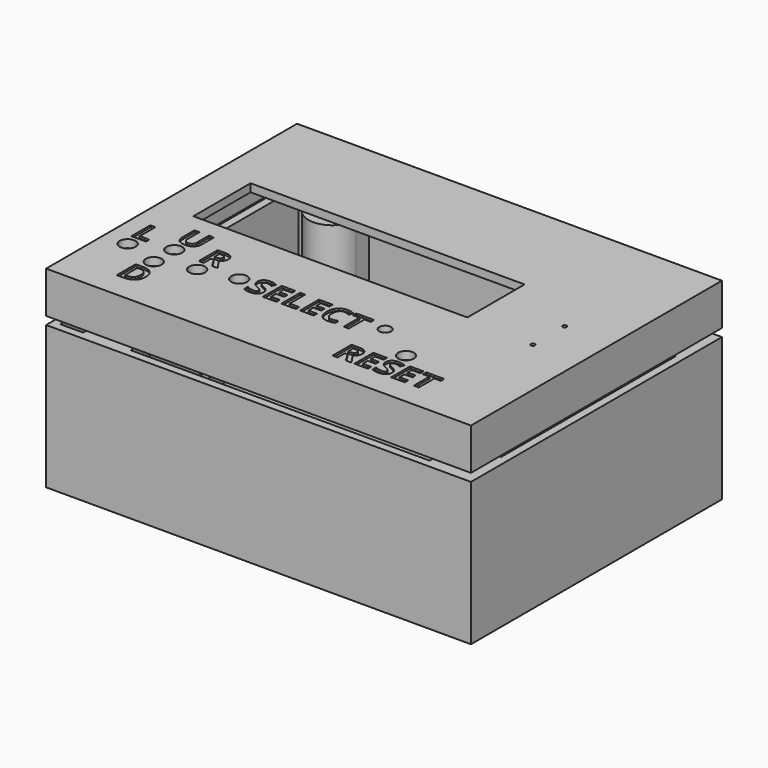
from build123d import *
from build123d import SkipClean  # not in build123d's __all__

# Parameters (mm, degrees)
F3_W         = 2
F3_H         = 5.75
F3_H_2       = 3.5
F3_R         = 2.1844
F3_H_3       = 10.1
F3_H_4       = 11
F4_DEPTH     = 2
F5_DEPTH     = 34
F6_START     = 3
F6_DEPTH     = 4
F7_START     = 3
F7_DEPTH     = 13
F8_START     = 32
F3_R_2       = 2
F8_DEPTH     = 2
F10_START    = 44.5
F9_W         = 107
F9_H         = 79
F9_R         = 0.5
F9_R_2       = 2.7813
F9_TEXT_SIZE = 8.3333333333
F10_DEPTH    = 2
F11_START    = 36
F11_DEPTH    = 8.5
F2_W         = 69
F2_H         = 18
F2_R         = 2
F2_R_2       = 1.5
F12_DEPTH    = 46.501
F13_START    = 46
F13_DEPTH    = 0.5
F14_R        = 2.75
F14_R_2      = 1.75
F15_DEPTH    = 7
F16_DEPTH    = 11.5


# Not quite as in the source:
# - after a boolean that leaves OpenCascade's solid faulty, fix() repairs it
# - a feature names something its author has since deleted; it is built from what else it names
# - Text() gives the source's letters only with a copy of the font that has no kerning and outlines rounded to 1/6400 em; it was checked with that copy


with BuildPart() as f4:
    # F3 (on Top) → F4 (new body)
    with BuildSketch(Plane.XY):
        Polygon((-51.5, 16.58), (-51.5, 37.5), (-45.8, 37.5), (-39.8, 37.5), (-33.8, 37.5), (41.5, 37.5), (47.5, 37.5), (51.5, 37.5), (51.5, 33.5), (51.5, 27.5), (51.5, -27.5), (51.5, -33.5), (51.5, -37.5), (47.4999999936, -37.5), (41.5, -37.5), (-33.8, -37.5), (-39.8, -37.5), (-45.8, -37.5), (-51.5, -37.5), (-51.5, -23.87), (-53.5, -23.87), (-53.5, -39.5), (53.5, -39.5), (53.5, 39.5), (-53.5, 39.5), (-53.5, 16.58), align=None)
        with Locations((-52.5, 3.605)):
            Rectangle(F3_W, F3_H)
        with Locations((-52.5, -11.12)):
            Rectangle(F3_W, F3_H_2)
        with BuildLine():
            Line((-45.8, 37.5), (-51.5, 37.5))
            Line((-51.5, 37.5), (-51.5, 16.58))
            Line((-51.5, 16.58), (-51.5, 6.48))
            Line((-51.5, 6.48), (-51.5, 0.73))
            Line((-51.5, 0.73), (-51.5, -9.37))
            Line((-51.5, -9.37), (-51.5, -12.87))
            Line((-51.5, -12.87), (-51.5, -23.87))
            Line((-51.5, -23.87), (-51.5, -37.5))
            Line((-51.5, -37.5), (-45.8, -37.5))
            Line((-45.8, -37.5), (-45.8, -33.5))
            ThreePointArc((-45.8, -33.5), (-39.8, -27.5), (-33.8, -33.5))
            Line((-33.8, -33.5), (-33.8, -37.5))
            Line((-33.8, -37.5), (41.5, -37.5))
            Line((41.5, -37.5), (41.5, -33.5))
            ThreePointArc((41.5, -33.5), (43.2573593129, -29.2573593129), (47.5, -27.5))
            Line((47.5, -27.5), (51.5, -27.5))
            Line((51.5, -27.5), (51.5, 27.5))
            Line((51.5, 27.5), (47.5, 27.5))
            ThreePointArc((47.5, 27.5), (43.2573593129, 29.2573593129), (41.5, 33.5))
            Line((41.5, 33.5), (41.5, 37.5))
            Line((41.5, 37.5), (-33.8, 37.5))
            Line((-33.8, 37.5), (-33.8, 33.5))
            ThreePointArc((-33.8, 33.5), (-39.8, 27.5), (-45.8, 33.5))
            Line((-45.8, 33.5), (-45.8, 37.5))
        make_face()
        with Locations((-35.56, -24.13)):
            Circle(F3_R, mode=Mode.SUBTRACT)
        with Locations((46.99, -24.13)):
            Circle(F3_R, mode=Mode.SUBTRACT)
        with Locations((-35.56, 24.13)):
            Circle(F3_R, mode=Mode.SUBTRACT)
        with Locations((-52.5, 11.53)):
            Rectangle(F3_W, F3_H_3)
        with Locations((-52.5, -4.32)):
            Rectangle(F3_W, F3_H_3)
        with Locations((-52.5, -18.37)):
            Rectangle(F3_W, F3_H_4)
        with BuildLine():
            Line((-45.8, 37.5), (-51.5, 37.5))
            Line((-51.5, 37.5), (-51.5, 16.58))
            Line((-51.5, 16.58), (-51.5, 6.48))
            Line((-51.5, 6.48), (-51.5, 0.73))
            Line((-51.5, 0.73), (-51.5, -9.37))
            Line((-51.5, -9.37), (-51.5, -12.87))
            Line((-51.5, -12.87), (-51.5, -23.87))
            Line((-51.5, -23.87), (-51.5, -37.5))
            Line((-51.5, -37.5), (-45.8, -37.5))
            Line((-45.8, -37.5), (-45.8, -33.5))
            ThreePointArc((-45.8, -33.5), (-39.8, -27.5), (-33.8, -33.5))
            Line((-33.8, -33.5), (-33.8, -37.5))
            Line((-33.8, -37.5), (41.5, -37.5))
            Line((41.5, -37.5), (41.5, -33.5))
            ThreePointArc((41.5, -33.5), (43.2573593129, -29.2573593129), (47.5, -27.5))
            Line((47.5, -27.5), (51.5, -27.5))
            Line((51.5, -27.5), (51.5, 27.5))
            Line((51.5, 27.5), (47.5, 27.5))
            ThreePointArc((47.5, 27.5), (43.2573593129, 29.2573593129), (41.5, 33.5))
            Line((41.5, 33.5), (41.5, 37.5))
            Line((41.5, 37.5), (-33.8, 37.5))
            Line((-33.8, 37.5), (-33.8, 33.5))
            ThreePointArc((-33.8, 33.5), (-39.8, 27.5), (-45.8, 33.5))
            Line((-45.8, 33.5), (-45.8, 37.5))
        make_face()
        with Locations((-35.56, -24.13)):
            Circle(F3_R, mode=Mode.SUBTRACT)
        with Locations((46.99, -24.13)):
            Circle(F3_R, mode=Mode.SUBTRACT)
        with Locations((-35.56, 24.13)):
            Circle(F3_R, mode=Mode.SUBTRACT)
        with BuildLine():
            Line((-45.8, -33.5), (-45.8, -37.5))
            Line((-45.8, -37.5), (-39.8, -37.5))
            Line((-39.8, -37.5), (-33.8, -37.5))
            Line((-33.8, -37.5), (-33.8, -33.5))
            ThreePointArc((-33.8, -33.5), (-39.8, -27.5), (-45.8, -33.5))
        make_face()
        with BuildLine():
            ThreePointArc((-35.8, -33.5), (-36.9715728753, -36.3284271247), (-39.8, -37.5))
            ThreePointArc((-39.8, -37.5), (-42.6284271247, -30.6715728753), (-35.8, -33.5))
        make_face(mode=Mode.SUBTRACT)
        with BuildLine():
            Line((-45.8, -33.5), (-45.8, -37.5))
            Line((-45.8, -37.5), (-39.8, -37.5))
            Line((-39.8, -37.5), (-33.8, -37.5))
            Line((-33.8, -37.5), (-33.8, -33.5))
            ThreePointArc((-33.8, -33.5), (-39.8, -27.5), (-45.8, -33.5))
        make_face()
        with BuildLine():
            ThreePointArc((-35.8, -33.5), (-36.9715728753, -36.3284271247), (-39.8, -37.5))
            ThreePointArc((-39.8, -37.5), (-42.6284271247, -30.6715728753), (-35.8, -33.5))
        make_face(mode=Mode.SUBTRACT)
        with BuildLine():
            Line((-45.8, 37.5), (-51.5, 37.5))
            Line((-51.5, 37.5), (-51.5, 16.58))
            Line((-51.5, 16.58), (-51.5, 6.48))
            Line((-51.5, 6.48), (-51.5, 0.73))
            Line((-51.5, 0.73), (-51.5, -9.37))
            Line((-51.5, -9.37), (-51.5, -12.87))
            Line((-51.5, -12.87), (-51.5, -23.87))
            Line((-51.5, -23.87), (-51.5, -37.5))
            Line((-51.5, -37.5), (-45.8, -37.5))
            Line((-45.8, -37.5), (-45.8, -33.5))
            ThreePointArc((-45.8, -33.5), (-39.8, -27.5), (-33.8, -33.5))
            Line((-33.8, -33.5), (-33.8, -37.5))
            Line((-33.8, -37.5), (41.5, -37.5))
            Line((41.5, -37.5), (41.5, -33.5))
            ThreePointArc((41.5, -33.5), (43.2573593129, -29.2573593129), (47.5, -27.5))
            Line((47.5, -27.5), (51.5, -27.5))
            Line((51.5, -27.5), (51.5, 27.5))
            Line((51.5, 27.5), (47.5, 27.5))
            ThreePointArc((47.5, 27.5), (43.2573593129, 29.2573593129), (41.5, 33.5))
            Line((41.5, 33.5), (41.5, 37.5))
            Line((41.5, 37.5), (-33.8, 37.5))
            Line((-33.8, 37.5), (-33.8, 33.5))
            ThreePointArc((-33.8, 33.5), (-39.8, 27.5), (-45.8, 33.5))
            Line((-45.8, 33.5), (-45.8, 37.5))
        make_face()
        with Locations((-35.56, -24.13)):
            Circle(F3_R, mode=Mode.SUBTRACT)
        with Locations((46.99, -24.13)):
            Circle(F3_R, mode=Mode.SUBTRACT)
        with Locations((-35.56, 24.13)):
            Circle(F3_R, mode=Mode.SUBTRACT)
        with BuildLine():
            Line((-39.8, 37.5), (-45.8, 37.5))
            Line((-45.8, 37.5), (-45.8, 33.5))
            ThreePointArc((-45.8, 33.5), (-39.8, 27.5), (-33.8, 33.5))
            Line((-33.8, 33.5), (-33.8, 37.5))
            Line((-33.8, 37.5), (-39.8, 37.5))
        make_face()
        with BuildLine():
            ThreePointArc((-35.8, 33.5), (-42.6284271247, 30.6715728753), (-39.8, 37.5))
            ThreePointArc((-39.8, 37.5), (-36.9715728753, 36.3284271247), (-35.8, 33.5))
        make_face(mode=Mode.SUBTRACT)
        with BuildLine():
            Line((47.5, 37.5), (41.5, 37.5))
            Line((41.5, 37.5), (41.5, 33.5))
            ThreePointArc((41.5, 33.5), (43.2573593129, 29.2573593129), (47.5, 27.5))
            Line((47.5, 27.5), (51.5, 27.5))
            Line((51.5, 27.5), (51.5, 33.5))
            ThreePointArc((51.5, 33.5), (44.6715728753, 30.6715728753), (47.5, 37.5))
        make_face()
        with BuildLine():
            Line((51.5, -33.5), (51.5, -27.5))
            Line((51.5, -27.5), (47.5, -27.5))
            ThreePointArc((47.5, -27.5), (43.2573593129, -29.2573593129), (41.5, -33.5))
            Line((41.5, -33.5), (41.5, -37.5))
            Line((41.5, -37.5), (47.4999999936, -37.5))
            ThreePointArc((47.4999999936, -37.5), (44.6715728775, -30.671572873), (51.5, -33.5))
        make_face()
        with BuildLine():
            Line((51.5, -37.5), (51.5, -33.5))
            ThreePointArc((51.5, -33.5), (50.3284271225, -36.328427127), (47.4999999936, -37.5))
            Line((47.4999999936, -37.5), (51.5, -37.5))
        make_face()
        with BuildLine():
            Line((-39.8, 37.5), (-45.8, 37.5))
            Line((-45.8, 37.5), (-45.8, 33.5))
            ThreePointArc((-45.8, 33.5), (-39.8, 27.5), (-33.8, 33.5))
            Line((-33.8, 33.5), (-33.8, 37.5))
            Line((-33.8, 37.5), (-39.8, 37.5))
        make_face()
        with BuildLine():
            ThreePointArc((-35.8, 33.5), (-42.6284271247, 30.6715728753), (-39.8, 37.5))
            ThreePointArc((-39.8, 37.5), (-36.9715728753, 36.3284271247), (-35.8, 33.5))
        make_face(mode=Mode.SUBTRACT)
        with BuildLine():
            Line((51.5, 37.5), (47.5, 37.5))
            ThreePointArc((47.5, 37.5), (50.3284271247, 36.3284271247), (51.5, 33.5))
            Line((51.5, 33.5), (51.5, 37.5))
        make_face()
    extrude(amount=-F4_DEPTH)

    # F3 (on Top) → F5 (join)
    with BuildSketch(Plane.XY):
        Polygon((-51.5, 16.58), (-51.5, 37.5), (-45.8, 37.5), (-39.8, 37.5), (-33.8, 37.5), (41.5, 37.5), (47.5, 37.5), (51.5, 37.5), (51.5, 33.5), (51.5, 27.5), (51.5, -27.5), (51.5, -33.5), (51.5, -37.5), (47.4999999936, -37.5), (41.5, -37.5), (-33.8, -37.5), (-39.8, -37.5), (-45.8, -37.5), (-51.5, -37.5), (-51.5, -23.87), (-53.5, -23.87), (-53.5, -39.5), (53.5, -39.5), (53.5, 39.5), (-53.5, 39.5), (-53.5, 16.58), align=None)
        with Locations((-52.5, -11.12)):
            Rectangle(F3_W, F3_H_2)
        with Locations((-52.5, 3.605)):
            Rectangle(F3_W, F3_H)
        with BuildLine():
            Line((-39.8, 37.5), (-45.8, 37.5))
            Line((-45.8, 37.5), (-45.8, 33.5))
            ThreePointArc((-45.8, 33.5), (-39.8, 27.5), (-33.8, 33.5))
            Line((-33.8, 33.5), (-33.8, 37.5))
            Line((-33.8, 37.5), (-39.8, 37.5))
        make_face()
        with BuildLine():
            ThreePointArc((-35.8, 33.5), (-42.6284271247, 30.6715728753), (-39.8, 37.5))
            ThreePointArc((-39.8, 37.5), (-36.9715728753, 36.3284271247), (-35.8, 33.5))
        make_face(mode=Mode.SUBTRACT)
        with BuildLine():
            Line((-39.8, 37.5), (-45.8, 37.5))
            Line((-45.8, 37.5), (-45.8, 33.5))
            ThreePointArc((-45.8, 33.5), (-39.8, 27.5), (-33.8, 33.5))
            Line((-33.8, 33.5), (-33.8, 37.5))
            Line((-33.8, 37.5), (-39.8, 37.5))
        make_face()
        with BuildLine():
            ThreePointArc((-35.8, 33.5), (-42.6284271247, 30.6715728753), (-39.8, 37.5))
            ThreePointArc((-39.8, 37.5), (-36.9715728753, 36.3284271247), (-35.8, 33.5))
        make_face(mode=Mode.SUBTRACT)
        with BuildLine():
            Line((47.5, 37.5), (41.5, 37.5))
            Line((41.5, 37.5), (41.5, 33.5))
            ThreePointArc((41.5, 33.5), (43.2573593129, 29.2573593129), (47.5, 27.5))
            Line((47.5, 27.5), (51.5, 27.5))
            Line((51.5, 27.5), (51.5, 33.5))
            ThreePointArc((51.5, 33.5), (44.6715728753, 30.6715728753), (47.5, 37.5))
        make_face()
        with BuildLine():
            Line((51.5, 37.5), (47.5, 37.5))
            ThreePointArc((47.5, 37.5), (50.3284271247, 36.3284271247), (51.5, 33.5))
            Line((51.5, 33.5), (51.5, 37.5))
        make_face()
        with BuildLine():
            Line((-45.8, -33.5), (-45.8, -37.5))
            Line((-45.8, -37.5), (-39.8, -37.5))
            Line((-39.8, -37.5), (-33.8, -37.5))
            Line((-33.8, -37.5), (-33.8, -33.5))
            ThreePointArc((-33.8, -33.5), (-39.8, -27.5), (-45.8, -33.5))
        make_face()
        with BuildLine():
            ThreePointArc((-35.8, -33.5), (-36.9715728753, -36.3284271247), (-39.8, -37.5))
            ThreePointArc((-39.8, -37.5), (-42.6284271247, -30.6715728753), (-35.8, -33.5))
        make_face(mode=Mode.SUBTRACT)
        with BuildLine():
            Line((-45.8, -33.5), (-45.8, -37.5))
            Line((-45.8, -37.5), (-39.8, -37.5))
            Line((-39.8, -37.5), (-33.8, -37.5))
            Line((-33.8, -37.5), (-33.8, -33.5))
            ThreePointArc((-33.8, -33.5), (-39.8, -27.5), (-45.8, -33.5))
        make_face()
        with BuildLine():
            ThreePointArc((-35.8, -33.5), (-36.9715728753, -36.3284271247), (-39.8, -37.5))
            ThreePointArc((-39.8, -37.5), (-42.6284271247, -30.6715728753), (-35.8, -33.5))
        make_face(mode=Mode.SUBTRACT)
        with BuildLine():
            Line((51.5, -37.5), (51.5, -33.5))
            ThreePointArc((51.5, -33.5), (50.3284271225, -36.328427127), (47.4999999936, -37.5))
            Line((47.4999999936, -37.5), (51.5, -37.5))
        make_face()
        with BuildLine():
            Line((51.5, -33.5), (51.5, -27.5))
            Line((51.5, -27.5), (47.5, -27.5))
            ThreePointArc((47.5, -27.5), (43.2573593129, -29.2573593129), (41.5, -33.5))
            Line((41.5, -33.5), (41.5, -37.5))
            Line((41.5, -37.5), (47.4999999936, -37.5))
            ThreePointArc((47.4999999936, -37.5), (44.6715728775, -30.671572873), (51.5, -33.5))
        make_face()
        with Locations((-52.5, 11.53)):
            Rectangle(F3_W, F3_H_3)
        with Locations((-52.5, -4.32)):
            Rectangle(F3_W, F3_H_3)
        with Locations((-52.5, -18.37)):
            Rectangle(F3_W, F3_H_4)
    with SkipClean():  # cleaning this boolean's faces spoils the solid; the shape is the same uncleaned
        extrude(amount=F5_DEPTH)

    # F3 (on Top) → F6 (cut)
    with BuildSketch(Plane.XY.offset(F6_START)):
        with Locations((-52.5, 11.53)):
            Rectangle(F3_W, F3_H_3)
        with Locations((-52.5, -4.32)):
            Rectangle(F3_W, F3_H_3)
    extrude(amount=F6_DEPTH, mode=Mode.SUBTRACT)

    add(f4.part.fix(), mode=Mode.REPLACE)

    # F3 (on Top) → F7 (cut)
    with BuildSketch(Plane.XY.offset(F7_START)):
        with Locations((-52.5, -18.37)):
            Rectangle(F3_W, F3_H_4)
    extrude(amount=F7_DEPTH, mode=Mode.SUBTRACT)

    # F3 (on Top) → F8 (join)
    with BuildSketch(Plane.XY.offset(F8_START)):
        with BuildLine():
            ThreePointArc((-35.8, 33.5), (-36.9715728753, 36.3284271247), (-39.8, 37.5))
            ThreePointArc((-39.8, 37.5), (-42.6284271247, 30.6715728753), (-35.8, 33.5))
        make_face()
        with Locations((-39.8, 33.5)):
            Circle(F3_R_2, mode=Mode.SUBTRACT)
        with BuildLine():
            ThreePointArc((-35.8, -33.5), (-42.6284271247, -30.6715728753), (-39.8, -37.5))
            ThreePointArc((-39.8, -37.5), (-36.9715728753, -36.3284271247), (-35.8, -33.5))
        make_face()
        with Locations((-39.8, -33.5)):
            Circle(F3_R_2, mode=Mode.SUBTRACT)
        with BuildLine():
            ThreePointArc((51.5, 33.5), (50.3284271247, 36.3284271247), (47.5, 37.5))
            ThreePointArc((47.5, 37.5), (44.6715728753, 30.6715728753), (51.5, 33.5))
        make_face()
        with Locations((47.5, 33.5)):
            Circle(F3_R_2, mode=Mode.SUBTRACT)
        with BuildLine():
            ThreePointArc((47.4999999936, -37.5), (50.3284271225, -36.328427127), (51.5, -33.5))
            ThreePointArc((51.5, -33.5), (44.6715728775, -30.671572873), (47.4999999936, -37.5))
        make_face()
        with Locations((47.5, -33.5)):
            Circle(F3_R_2, mode=Mode.SUBTRACT)
    extrude(amount=F8_DEPTH)


with BuildPart() as f10:
    # F9 (on Top) → F10 (new body)
    with BuildSketch(Plane.XY.offset(F10_START)):
        Rectangle(F9_W, F9_H)
        Polygon((-51.5, -37.5), (-51.5, 37.5), (-45.8, 37.5), (-33.8, 37.5), (41.5, 37.5), (51.5, 37.5), (51.5, 27.5), (51.5, -27.5), (51.5, -37.5), (41.5, -37.5), (-33.8, -37.5), (-45.8, -37.5), align=None, mode=Mode.SUBTRACT)
        with BuildLine():
            Line((-45.8, 37.5), (-51.5, 37.5))
            Line((-51.5, 37.5), (-51.5, -37.5))
            Line((-51.5, -37.5), (-45.8, -37.5))
            Line((-45.8, -37.5), (-45.8, -33.5))
            ThreePointArc((-45.8, -33.5), (-44.4131605218, -29.6634976867), (-40.89375, -27.6005329955))
            Line((-40.89375, -27.6005329955), (-40.89375, -27.05078125))
            Line((-40.89375, -27.05078125), (-39.0265625, -27.05078125))
            add(Edge.make_bspline(
                [(-39.0265625, -27.05078125), (-37.56953125, -27.05078125), (-36.7635416667, -27.8196614583)],
                knots=[0, 0, 0, 1, 1, 1], degree=2))
            add(Edge.make_bspline(
                [(-36.7635416667, -27.8196614583), (-36.3660320041, -28.1988689798), (-36.1645719371, -28.7267764771)],
                knots=[0, 0, 0, 0.493194541, 0.493194541, 0.493194541], degree=2))
            ThreePointArc((-36.1645719371, -28.7267764771), (-34.4235435286, -30.8365969492), (-33.8, -33.5))
            Line((-33.8, -33.5), (-33.8, -37.5))
            Line((-33.8, -37.5), (41.5, -37.5))
            Line((41.5, -37.5), (41.5, -33.5))
            ThreePointArc((41.5, -33.5), (43.2573593129, -29.2573593129), (47.5, -27.5))
            Line((47.5, -27.5), (51.5, -27.5))
            Line((51.5, -27.5), (51.5, 27.5))
            Line((51.5, 27.5), (47.5, 27.5))
            ThreePointArc((47.5, 27.5), (43.2573593129, 29.2573593129), (41.5, 33.5))
            Line((41.5, 33.5), (41.5, 37.5))
            Line((41.5, 37.5), (-33.8, 37.5))
            Line((-33.8, 37.5), (-33.8, 33.5))
            ThreePointArc((-33.8, 33.5), (-39.8, 27.5), (-45.8, 33.5))
            Line((-45.8, 33.5), (-45.8, 37.5))
        make_face()
        Polygon((-45.3384114583, -18.25), (-49.012890625, -18.25), (-49.012890625, -12.30078125), (-47.751171875, -12.30078125), (-47.751171875, -17.2083333333), (-45.3384114583, -17.2083333333), align=None, mode=Mode.SUBTRACT)
        with BuildLine():
            Line((-30.1196614583, -15.9674479167), (-30.790234375, -15.9674479167))
            Line((-30.790234375, -15.9674479167), (-30.790234375, -18.25))
            Line((-30.790234375, -18.25), (-32.051953125, -18.25))
            Line((-32.051953125, -18.25), (-32.051953125, -12.30078125))
            Line((-32.051953125, -12.30078125), (-30.3188802083, -12.30078125))
            add(Edge.make_bspline(
                [(-30.3188802083, -12.30078125), (-29.1053385417, -12.30078125), (-28.5239583333, -12.7421875)],
                knots=[0, 0, 0, 1, 1, 1], degree=2))
            add(Edge.make_bspline(
                [(-28.5239583333, -12.7421875), (-27.942578125, -13.18359375), (-27.942578125, -14.0833333333)],
                knots=[0, 0, 0, 1, 1, 1], degree=2))
            add(Edge.make_bspline(
                [(-27.942578125, -14.0833333333), (-27.942578125, -14.6080729167), (-28.2309895833, -15.0169270833)],
                knots=[0, 0, 0, 1, 1, 1], degree=2))
            add(Edge.make_bspline(
                [(-28.2309895833, -15.0169270833), (-28.5194010417, -15.42578125), (-29.0493489583, -15.6575520833)],
                knots=[0, 0, 0, 1, 1, 1], degree=2))
            add(Edge.make_bspline(
                [(-29.0493489583, -15.6575520833), (-27.7055989583, -17.6640625), (-27.2993489583, -18.25)],
                knots=[0, 0, 0, 1, 1, 1], degree=2))
            Line((-27.2993489583, -18.25), (-28.6990885417, -18.25))
            Line((-28.6990885417, -18.25), (-30.1196614583, -15.9674479167))
        make_face(mode=Mode.SUBTRACT)
        with BuildLine():
            Line((-37.2622395833, -8.55078125), (-36.0044270833, -8.55078125))
            Line((-36.0044270833, -8.55078125), (-36.0044270833, -12.3997395833))
            add(Edge.make_bspline(
                [(-36.0044270833, -12.3997395833), (-36.0044270833, -13.0598958333), (-36.2993489583, -13.5559895833)],
                knots=[0, 0, 0, 1, 1, 1], degree=2))
            add(Edge.make_bspline(
                [(-36.2993489583, -13.5559895833), (-36.5942708333, -14.0520833333), (-37.1522135417, -14.3170572917)],
                knots=[0, 0, 0, 1, 1, 1], degree=2))
            add(Edge.make_bspline(
                [(-37.1522135417, -14.3170572917), (-37.71015625, -14.58203125), (-38.4705729167, -14.58203125)],
                knots=[0, 0, 0, 1, 1, 1], degree=2))
            add(Edge.make_bspline(
                [(-38.4705729167, -14.58203125), (-39.6177083333, -14.58203125), (-40.2524739583, -13.9934895833)],
                knots=[0, 0, 0, 1, 1, 1], degree=2))
            add(Edge.make_bspline(
                [(-40.2524739583, -13.9934895833), (-40.8872395833, -13.4049479167), (-40.8872395833, -12.3841145833)],
                knots=[0, 0, 0, 1, 1, 1], degree=2))
            Line((-40.8872395833, -12.3841145833), (-40.8872395833, -8.55078125))
            Line((-40.8872395833, -8.55078125), (-39.6307291667, -8.55078125))
            Line((-39.6307291667, -8.55078125), (-39.6307291667, -12.1927083333))
            add(Edge.make_bspline(
                [(-39.6307291667, -12.1927083333), (-39.6307291667, -12.8802083333), (-39.3540364583, -13.2018229167)],
                knots=[0, 0, 0, 1, 1, 1], degree=2))
            add(Edge.make_bspline(
                [(-39.3540364583, -13.2018229167), (-39.07734375, -13.5234375), (-38.4380208333, -13.5234375)],
                knots=[0, 0, 0, 1, 1, 1], degree=2))
            add(Edge.make_bspline(
                [(-38.4380208333, -13.5234375), (-37.81953125, -13.5234375), (-37.5408854167, -13.1998697917)],
                knots=[0, 0, 0, 1, 1, 1], degree=2))
            add(Edge.make_bspline(
                [(-37.5408854167, -13.1998697917), (-37.2622395833, -12.8763020833), (-37.2622395833, -12.1848958333)],
                knots=[0, 0, 0, 1, 1, 1], degree=2))
            Line((-37.2622395833, -12.1848958333), (-37.2622395833, -8.55078125))
        make_face(mode=Mode.SUBTRACT)
        with BuildLine():
            add(Edge.make_bspline(
                [(-14.098828125, -19.615234375), (-13.7895833333, -20.015625), (-13.7895833333, -20.59765625)],
                knots=[0, 0, 0, 1, 1, 1], degree=2))
            add(Edge.make_bspline(
                [(-13.7895833333, -20.59765625), (-13.7895833333, -21.4036458333), (-14.3696614583, -21.8678385417)],
                knots=[0, 0, 0, 1, 1, 1], degree=2))
            add(Edge.make_bspline(
                [(-14.3696614583, -21.8678385417), (-14.9497395833, -22.33203125), (-15.9822916667, -22.33203125)],
                knots=[0, 0, 0, 1, 1, 1], degree=2))
            add(Edge.make_bspline(
                [(-15.9822916667, -22.33203125), (-16.9354166667, -22.33203125), (-17.6671875, -21.97265625)],
                knots=[0, 0, 0, 1, 1, 1], degree=2))
            Line((-17.6671875, -21.97265625), (-17.6671875, -20.80078125))
            add(Edge.make_bspline(
                [(-17.6671875, -20.80078125), (-17.065625, -21.0703125), (-16.6483072917, -21.1796875)],
                knots=[0, 0, 0, 1, 1, 1], degree=2))
            add(Edge.make_bspline(
                [(-16.6483072917, -21.1796875), (-16.2309895833, -21.2890625), (-15.8846354167, -21.2890625)],
                knots=[0, 0, 0, 1, 1, 1], degree=2))
            add(Edge.make_bspline(
                [(-15.8846354167, -21.2890625), (-15.4705729167, -21.2890625), (-15.2485677083, -21.130859375)],
                knots=[0, 0, 0, 1, 1, 1], degree=2))
            add(Edge.make_bspline(
                [(-15.2485677083, -21.130859375), (-15.0265625, -20.97265625), (-15.0265625, -20.6588541667)],
                knots=[0, 0, 0, 1, 1, 1], degree=2))
            add(Edge.make_bspline(
                [(-15.0265625, -20.6588541667), (-15.0265625, -20.484375), (-15.12421875, -20.34765625)],
                knots=[0, 0, 0, 1, 1, 1], degree=2))
            add(Edge.make_bspline(
                [(-15.12421875, -20.34765625), (-15.221875, -20.2109375), (-15.411328125, -20.0852864583)],
                knots=[0, 0, 0, 1, 1, 1], degree=2))
            add(Edge.make_bspline(
                [(-15.411328125, -20.0852864583), (-15.60078125, -19.9596354167), (-16.1828125, -19.6822916667)],
                knots=[0, 0, 0, 1, 1, 1], degree=2))
            add(Edge.make_bspline(
                [(-16.1828125, -19.6822916667), (-16.7270833333, -19.42578125), (-16.9998697917, -19.1901041667)],
                knots=[0, 0, 0, 1, 1, 1], degree=2))
            add(Edge.make_bspline(
                [(-16.9998697917, -19.1901041667), (-17.27265625, -18.9544270833), (-17.4354166667, -18.640625)],
                knots=[0, 0, 0, 1, 1, 1], degree=2))
            add(Edge.make_bspline(
                [(-17.4354166667, -18.640625), (-17.5981770833, -18.3268229167), (-17.5981770833, -17.9088541667)],
                knots=[0, 0, 0, 1, 1, 1], degree=2))
            add(Edge.make_bspline(
                [(-17.5981770833, -17.9088541667), (-17.5981770833, -17.1184895833), (-17.0630208333, -16.6673177083)],
                knots=[0, 0, 0, 1, 1, 1], degree=2))
            add(Edge.make_bspline(
                [(-17.0630208333, -16.6673177083), (-16.5278645833, -16.2161458333), (-15.5838541667, -16.2161458333)],
                knots=[0, 0, 0, 1, 1, 1], degree=2))
            add(Edge.make_bspline(
                [(-15.5838541667, -16.2161458333), (-15.1203125, -16.2161458333), (-14.6990885417, -16.3255208333)],
                knots=[0, 0, 0, 1, 1, 1], degree=2))
            add(Edge.make_bspline(
                [(-14.6990885417, -16.3255208333), (-14.2778645833, -16.4348958333), (-13.8182291667, -16.6341145833)],
                knots=[0, 0, 0, 1, 1, 1], degree=2))
            Line((-13.8182291667, -16.6341145833), (-14.2244791667, -17.6158854167))
            add(Edge.make_bspline(
                [(-14.2244791667, -17.6158854167), (-14.7010416667, -17.4205729167), (-15.0122395833, -17.3430989583)],
                knots=[0, 0, 0, 1, 1, 1], degree=2))
            add(Edge.make_bspline(
                [(-15.0122395833, -17.3430989583), (-15.3234375, -17.265625), (-15.62421875, -17.265625)],
                knots=[0, 0, 0, 1, 1, 1], degree=2))
            add(Edge.make_bspline(
                [(-15.62421875, -17.265625), (-15.9822916667, -17.265625), (-16.1736979167, -17.4322916667)],
                knots=[0, 0, 0, 1, 1, 1], degree=2))
            add(Edge.make_bspline(
                [(-16.1736979167, -17.4322916667), (-16.3651041667, -17.5989583333), (-16.3651041667, -17.8671875)],
                knots=[0, 0, 0, 1, 1, 1], degree=2))
            add(Edge.make_bspline(
                [(-16.3651041667, -17.8671875), (-16.3651041667, -18.0338541667), (-16.2876302083, -18.158203125)],
                knots=[0, 0, 0, 1, 1, 1], degree=2))
            add(Edge.make_bspline(
                [(-16.2876302083, -18.158203125), (-16.21015625, -18.2825520833), (-16.0415364583, -18.3984375)],
                knots=[0, 0, 0, 1, 1, 1], degree=2))
            add(Edge.make_bspline(
                [(-16.0415364583, -18.3984375), (-15.8729166667, -18.5143229167), (-15.2427083333, -18.8151041667)],
                knots=[0, 0, 0, 1, 1, 1], degree=2))
            add(Edge.make_bspline(
                [(-15.2427083333, -18.8151041667), (-14.4080729167, -19.21484375), (-14.098828125, -19.615234375)],
                knots=[0, 0, 0, 1, 1, 1], degree=2))
        make_face(mode=Mode.SUBTRACT)
        Polygon((-9.2856770833, -21.2083333333), (-9.2856770833, -22.25), (-12.7114583333, -22.25), (-12.7114583333, -16.30078125), (-9.2856770833, -16.30078125), (-9.2856770833, -17.3346354167), (-11.4497395833, -17.3346354167), (-11.4497395833, -18.640625), (-9.4354166667, -18.640625), (-9.4354166667, -19.6744791667), (-11.4497395833, -19.6744791667), (-11.4497395833, -21.2083333333), align=None, mode=Mode.SUBTRACT)
        Polygon((-4.3703125, -22.25), (-8.0447916667, -22.25), (-8.0447916667, -16.30078125), (-6.7830729167, -16.30078125), (-6.7830729167, -21.2083333333), (-4.3703125, -21.2083333333), align=None, mode=Mode.SUBTRACT)
        Polygon((0.0893229167, -21.2083333333), (0.0893229167, -22.25), (-3.3364583333, -22.25), (-3.3364583333, -16.30078125), (0.0893229167, -16.30078125), (0.0893229167, -17.3346354167), (-2.0747395833, -17.3346354167), (-2.0747395833, -18.640625), (-0.0604166667, -18.640625), (-0.0604166667, -19.6744791667), (-2.0747395833, -19.6744791667), (-2.0747395833, -21.2083333333), align=None, mode=Mode.SUBTRACT)
        with BuildLine():
            Line((15.5893229167, -30.9674479167), (14.91875, -30.9674479167))
            Line((14.91875, -30.9674479167), (14.91875, -33.25))
            Line((14.91875, -33.25), (13.65703125, -33.25))
            Line((13.65703125, -33.25), (13.65703125, -27.30078125))
            Line((13.65703125, -27.30078125), (15.3901041667, -27.30078125))
            add(Edge.make_bspline(
                [(15.3901041667, -27.30078125), (16.6036458333, -27.30078125), (17.1850260417, -27.7421875)],
                knots=[0, 0, 0, 1, 1, 1], degree=2))
            add(Edge.make_bspline(
                [(17.1850260417, -27.7421875), (17.76640625, -28.18359375), (17.76640625, -29.0833333333)],
                knots=[0, 0, 0, 1, 1, 1], degree=2))
            add(Edge.make_bspline(
                [(17.76640625, -29.0833333333), (17.76640625, -29.6080729167), (17.4779947917, -30.0169270833)],
                knots=[0, 0, 0, 1, 1, 1], degree=2))
            add(Edge.make_bspline(
                [(17.4779947917, -30.0169270833), (17.1895833333, -30.42578125), (16.6596354167, -30.6575520833)],
                knots=[0, 0, 0, 1, 1, 1], degree=2))
            add(Edge.make_bspline(
                [(16.6596354167, -30.6575520833), (18.0033854167, -32.6640625), (18.4096354167, -33.25)],
                knots=[0, 0, 0, 1, 1, 1], degree=2))
            Line((18.4096354167, -33.25), (17.0098958333, -33.25))
            Line((17.0098958333, -33.25), (15.5893229167, -30.9674479167))
        make_face(mode=Mode.SUBTRACT)
        Polygon((22.5841145833, -32.2083333333), (22.5841145833, -33.25), (19.1583333333, -33.25), (19.1583333333, -27.30078125), (22.5841145833, -27.30078125), (22.5841145833, -28.3346354167), (20.4200520833, -28.3346354167), (20.4200520833, -29.640625), (22.434375, -29.640625), (22.434375, -30.6744791667), (20.4200520833, -30.6744791667), (20.4200520833, -32.2083333333), align=None, mode=Mode.SUBTRACT)
        with BuildLine():
            add(Edge.make_bspline(
                [(27.0274739583, -30.615234375), (27.33671875, -31.015625), (27.33671875, -31.59765625)],
                knots=[0, 0, 0, 1, 1, 1], degree=2))
            add(Edge.make_bspline(
                [(27.33671875, -31.59765625), (27.33671875, -32.4036458333), (26.756640625, -32.8678385417)],
                knots=[0, 0, 0, 1, 1, 1], degree=2))
            add(Edge.make_bspline(
                [(26.756640625, -32.8678385417), (26.1765625, -33.33203125), (25.1440104167, -33.33203125)],
                knots=[0, 0, 0, 1, 1, 1], degree=2))
            add(Edge.make_bspline(
                [(25.1440104167, -33.33203125), (24.1908854167, -33.33203125), (23.4591145833, -32.97265625)],
                knots=[0, 0, 0, 1, 1, 1], degree=2))
            Line((23.4591145833, -32.97265625), (23.4591145833, -31.80078125))
            add(Edge.make_bspline(
                [(23.4591145833, -31.80078125), (24.0606770833, -32.0703125), (24.4779947917, -32.1796875)],
                knots=[0, 0, 0, 1, 1, 1], degree=2))
            add(Edge.make_bspline(
                [(24.4779947917, -32.1796875), (24.8953125, -32.2890625), (25.2416666667, -32.2890625)],
                knots=[0, 0, 0, 1, 1, 1], degree=2))
            add(Edge.make_bspline(
                [(25.2416666667, -32.2890625), (25.6557291667, -32.2890625), (25.877734375, -32.130859375)],
                knots=[0, 0, 0, 1, 1, 1], degree=2))
            add(Edge.make_bspline(
                [(25.877734375, -32.130859375), (26.0997395833, -31.97265625), (26.0997395833, -31.6588541667)],
                knots=[0, 0, 0, 1, 1, 1], degree=2))
            add(Edge.make_bspline(
                [(26.0997395833, -31.6588541667), (26.0997395833, -31.484375), (26.0020833333, -31.34765625)],
                knots=[0, 0, 0, 1, 1, 1], degree=2))
            add(Edge.make_bspline(
                [(26.0020833333, -31.34765625), (25.9044270833, -31.2109375), (25.7149739583, -31.0852864583)],
                knots=[0, 0, 0, 1, 1, 1], degree=2))
            add(Edge.make_bspline(
                [(25.7149739583, -31.0852864583), (25.5255208333, -30.9596354167), (24.9434895833, -30.6822916667)],
                knots=[0, 0, 0, 1, 1, 1], degree=2))
            add(Edge.make_bspline(
                [(24.9434895833, -30.6822916667), (24.39921875, -30.42578125), (24.1264322917, -30.1901041667)],
                knots=[0, 0, 0, 1, 1, 1], degree=2))
            add(Edge.make_bspline(
                [(24.1264322917, -30.1901041667), (23.8536458333, -29.9544270833), (23.6908854167, -29.640625)],
                knots=[0, 0, 0, 1, 1, 1], degree=2))
            add(Edge.make_bspline(
                [(23.6908854167, -29.640625), (23.528125, -29.3268229167), (23.528125, -28.9088541667)],
                knots=[0, 0, 0, 1, 1, 1], degree=2))
            add(Edge.make_bspline(
                [(23.528125, -28.9088541667), (23.528125, -28.1184895833), (24.06328125, -27.6673177083)],
                knots=[0, 0, 0, 1, 1, 1], degree=2))
            add(Edge.make_bspline(
                [(24.06328125, -27.6673177083), (24.5984375, -27.2161458333), (25.5424479167, -27.2161458333)],
                knots=[0, 0, 0, 1, 1, 1], degree=2))
            add(Edge.make_bspline(
                [(25.5424479167, -27.2161458333), (26.0059895833, -27.2161458333), (26.4272135417, -27.3255208333)],
                knots=[0, 0, 0, 1, 1, 1], degree=2))
            add(Edge.make_bspline(
                [(26.4272135417, -27.3255208333), (26.8484375, -27.4348958333), (27.3080729167, -27.6341145833)],
                knots=[0, 0, 0, 1, 1, 1], degree=2))
            Line((27.3080729167, -27.6341145833), (26.9018229167, -28.6158854167))
            add(Edge.make_bspline(
                [(26.9018229167, -28.6158854167), (26.4252604167, -28.4205729167), (26.1140625, -28.3430989583)],
                knots=[0, 0, 0, 1, 1, 1], degree=2))
            add(Edge.make_bspline(
                [(26.1140625, -28.3430989583), (25.8028645833, -28.265625), (25.5020833333, -28.265625)],
                knots=[0, 0, 0, 1, 1, 1], degree=2))
            add(Edge.make_bspline(
                [(25.5020833333, -28.265625), (25.1440104167, -28.265625), (24.9526041667, -28.4322916667)],
                knots=[0, 0, 0, 1, 1, 1], degree=2))
            add(Edge.make_bspline(
                [(24.9526041667, -28.4322916667), (24.7611979167, -28.5989583333), (24.7611979167, -28.8671875)],
                knots=[0, 0, 0, 1, 1, 1], degree=2))
            add(Edge.make_bspline(
                [(24.7611979167, -28.8671875), (24.7611979167, -29.0338541667), (24.838671875, -29.158203125)],
                knots=[0, 0, 0, 1, 1, 1], degree=2))
            add(Edge.make_bspline(
                [(24.838671875, -29.158203125), (24.9161458333, -29.2825520833), (25.084765625, -29.3984375)],
                knots=[0, 0, 0, 1, 1, 1], degree=2))
            add(Edge.make_bspline(
                [(25.084765625, -29.3984375), (25.2533854167, -29.5143229167), (25.88359375, -29.8151041667)],
                knots=[0, 0, 0, 1, 1, 1], degree=2))
            add(Edge.make_bspline(
                [(25.88359375, -29.8151041667), (26.7182291667, -30.21484375), (27.0274739583, -30.615234375)],
                knots=[0, 0, 0, 1, 1, 1], degree=2))
        make_face(mode=Mode.SUBTRACT)
        Polygon((31.840625, -32.2083333333), (31.840625, -33.25), (28.41484375, -33.25), (28.41484375, -27.30078125), (31.840625, -27.30078125), (31.840625, -28.3346354167), (29.6765625, -28.3346354167), (29.6765625, -29.640625), (31.6908854167, -29.640625), (31.6908854167, -30.6744791667), (29.6765625, -30.6744791667), (29.6765625, -32.2083333333), align=None, mode=Mode.SUBTRACT)
        Polygon((35.3770833333, -28.3502604167), (35.3770833333, -33.25), (34.1153645833, -33.25), (34.1153645833, -28.3502604167), (32.4994791667, -28.3502604167), (32.4994791667, -27.30078125), (36.9916666667, -27.30078125), (36.9916666667, -28.3502604167), align=None, mode=Mode.SUBTRACT)
        with BuildLine():
            add(Edge.make_bspline(
                [(4.5203125, -17.3834635417), (4.1830729167, -17.265625), (3.8575520833, -17.265625)],
                knots=[0, 0, 0, 1, 1, 1], degree=2))
            add(Edge.make_bspline(
                [(3.8575520833, -17.265625), (3.1453125, -17.265625), (2.7546875, -17.80078125)],
                knots=[0, 0, 0, 1, 1, 1], degree=2))
            add(Edge.make_bspline(
                [(2.7546875, -17.80078125), (2.3640625, -18.3359375), (2.3640625, -19.2916666667)],
                knots=[0, 0, 0, 1, 1, 1], degree=2))
            add(Edge.make_bspline(
                [(2.3640625, -19.2916666667), (2.3640625, -21.28125), (3.8575520833, -21.28125)],
                knots=[0, 0, 0, 1, 1, 1], degree=2))
            add(Edge.make_bspline(
                [(3.8575520833, -21.28125), (4.4838541667, -21.28125), (5.3744791667, -20.96875)],
                knots=[0, 0, 0, 1, 1, 1], degree=2))
            Line((5.3744791667, -20.96875), (5.3744791667, -22.0260416667))
            add(Edge.make_bspline(
                [(5.3744791667, -22.0260416667), (4.6427083333, -22.33203125), (3.7390625, -22.33203125)],
                knots=[0, 0, 0, 1, 1, 1], degree=2))
            add(Edge.make_bspline(
                [(3.7390625, -22.33203125), (2.4408854167, -22.33203125), (1.7533854167, -21.5442708333)],
                knots=[0, 0, 0, 1, 1, 1], degree=2))
            add(Edge.make_bspline(
                [(1.7533854167, -21.5442708333), (1.0658854167, -20.7565104167), (1.0658854167, -19.2838541667)],
                knots=[0, 0, 0, 1, 1, 1], degree=2))
            add(Edge.make_bspline(
                [(1.0658854167, -19.2838541667), (1.0658854167, -18.35546875), (1.4037760417, -17.6575520833)],
                knots=[0, 0, 0, 1, 1, 1], degree=2))
            add(Edge.make_bspline(
                [(1.4037760417, -17.6575520833), (1.7416666667, -16.9596354167), (2.3744791667, -16.587890625)],
                knots=[0, 0, 0, 1, 1, 1], degree=2))
            add(Edge.make_bspline(
                [(2.3744791667, -16.587890625), (3.0072916667, -16.2161458333), (3.8575520833, -16.2161458333)],
                knots=[0, 0, 0, 1, 1, 1], degree=2))
            add(Edge.make_bspline(
                [(3.8575520833, -16.2161458333), (4.7234375, -16.2161458333), (5.5984375, -16.6341145833)],
                knots=[0, 0, 0, 1, 1, 1], degree=2))
            Line((5.5984375, -16.6341145833), (5.1921875, -17.66015625))
            add(Edge.make_bspline(
                [(5.1921875, -17.66015625), (4.8575520833, -17.5013020833), (4.5203125, -17.3834635417)],
                knots=[0, 0, 0, 1, 1, 1], degree=2))
        make_face(mode=Mode.SUBTRACT)
        Polygon((8.9356770833, -17.3502604167), (8.9356770833, -22.25), (7.6739583333, -22.25), (7.6739583333, -17.3502604167), (6.0580729167, -17.3502604167), (6.0580729167, -16.30078125), (10.5502604167, -16.30078125), (10.5502604167, -17.3502604167), align=None, mode=Mode.SUBTRACT)
        with Locations((41.5, -5)):
            Circle(F9_R, mode=Mode.SUBTRACT)
        with Locations((41.5, 5)):
            Circle(F9_R, mode=Mode.SUBTRACT)
        with BuildLine():
            Line((-33.8, 37.5), (-45.8, 37.5))
            Line((-45.8, 37.5), (-45.8, 33.5))
            ThreePointArc((-45.8, 33.5), (-39.8, 27.5), (-33.8, 33.5))
            Line((-33.8, 33.5), (-33.8, 37.5))
        make_face()
        with Locations((-39.8, 33.5)):
            Circle(F9_R_2, mode=Mode.SUBTRACT)
        with BuildLine():
            Line((41.5, -33.5), (41.5, -37.5))
            Line((41.5, -37.5), (51.5, -37.5))
            Line((51.5, -37.5), (51.5, -27.5))
            Line((51.5, -27.5), (47.5, -27.5))
            ThreePointArc((47.5, -27.5), (43.2573593129, -29.2573593129), (41.5, -33.5))
        make_face()
        with Locations((47.5, -33.5)):
            Circle(F9_R_2, mode=Mode.SUBTRACT)
        with BuildLine():
            Line((51.5, 37.5), (41.5, 37.5))
            Line((41.5, 37.5), (41.5, 33.5))
            ThreePointArc((41.5, 33.5), (43.2573593129, 29.2573593129), (47.5, 27.5))
            Line((47.5, 27.5), (51.5, 27.5))
            Line((51.5, 27.5), (51.5, 37.5))
        make_face()
        with Locations((47.5, 33.5)):
            Circle(F9_R_2, mode=Mode.SUBTRACT)
        with BuildLine():
            Line((-45.8, -33.5), (-45.8, -37.5))
            Line((-45.8, -37.5), (-33.8, -37.5))
            Line((-33.8, -37.5), (-33.8, -33.5))
            ThreePointArc((-33.8, -33.5), (-34.4235435286, -30.8365969492), (-36.1645719371, -28.7267764771))
            add(Edge.make_bspline(
                [(-36.1645719371, -28.7267764771), (-35.9575520833, -29.2692528821), (-35.9575520833, -29.96875)],
                knots=[0.493194541, 0.493194541, 0.493194541, 1, 1, 1], degree=2))
            add(Edge.make_bspline(
                [(-35.9575520833, -29.96875), (-35.9575520833, -31.4375), (-36.794140625, -32.21875)],
                knots=[0, 0, 0, 1, 1, 1], degree=2))
            add(Edge.make_bspline(
                [(-36.794140625, -32.21875), (-36.97723038, -32.3897287595), (-37.1958371755, -32.5232883366)],
                knots=[0, 0, 0, 0.2188528121, 0.2188528121, 0.2188528121], degree=2))
            ThreePointArc((-37.1958371755, -32.5232883366), (-37.0633425722, -33.0036777125), (-37.0187, -33.5))
            ThreePointArc((-37.0187, -33.5), (-41.3319240867, -35.8213871462), (-40.89375, -30.9427865503))
            Line((-40.89375, -30.9427865503), (-40.89375, -27.6005329955))
            ThreePointArc((-40.89375, -27.6005329955), (-44.4131605218, -29.6634976867), (-45.8, -33.5))
        make_face()
        with Locations((47.5, -33.5)):
            Circle(F9_R_2)
        with Locations((-39.8, 33.5)):
            Circle(F9_R_2)
        with Locations((47.5, 33.5)):
            Circle(F9_R_2)
        with Locations((-32.8006510417, -18.25)):
            Text('R', F9_TEXT_SIZE, font='Open Sans', font_style=FontStyle.BOLD, text_align=(TextAlign.LEFT, TextAlign.BOTTOM))
        with BuildLine():
            Line((-40.89375, -33), (-40.89375, -30.9427865503))
            ThreePointArc((-40.89375, -30.9427865503), (-41.3319240867, -35.8213871462), (-37.0187, -33.5))
            ThreePointArc((-37.0187, -33.5), (-37.0633425722, -33.0036777125), (-37.1958371755, -32.5232883366))
            add(Edge.make_bspline(
                [(-37.1958371755, -32.5232883366), (-37.9761062608, -33), (-39.2088541667, -33)],
                knots=[0.2188528121, 0.2188528121, 0.2188528121, 1, 1, 1], degree=2))
            Line((-39.2088541667, -33), (-40.89375, -33))
        make_face()
        with Locations((-41.5955729167, -14.5)):
            Text('U', F9_TEXT_SIZE, font='Open Sans', font_style=FontStyle.BOLD, text_align=(TextAlign.LEFT, TextAlign.BOTTOM))
        with Locations((12.9083333333, -33.25)):
            Text('RESET', F9_TEXT_SIZE, font='Open Sans', font_style=FontStyle.BOLD, text_align=(TextAlign.LEFT, TextAlign.BOTTOM))
        with BuildLine():
            ThreePointArc((-36.1645719371, -28.7267764771), (-38.409986353, -27.6632318822), (-40.89375, -27.6005329955))
            Line((-40.89375, -27.6005329955), (-40.89375, -30.9427865503))
            ThreePointArc((-40.89375, -30.9427865503), (-40.2756669705, -30.7596769126), (-39.63203125, -30.723776632))
            Line((-39.63203125, -30.723776632), (-39.63203125, -28.0846354167))
            Line((-39.63203125, -28.0846354167), (-38.9614583333, -28.0846354167))
            add(Edge.make_bspline(
                [(-37.26875, -30.0013020833), (-37.26875, -28.0846354167), (-38.9614583333, -28.0846354167)],
                knots=[0, 0, 0, 1, 1, 1], degree=2))
            add(Edge.make_bspline(
                [(-37.8120490306, -31.5548314641), (-37.26875, -31.0697019319), (-37.26875, -30.0013020833)],
                knots=[0.4540711353, 0.4540711353, 0.4540711353, 1, 1, 1], degree=2))
            ThreePointArc((-37.8120490306, -31.5548314641), (-37.4534377373, -32.0069242359), (-37.1958371755, -32.5232883366))
            add(Edge.make_bspline(
                [(-36.794140625, -32.21875), (-36.97723038, -32.3897287595), (-37.1958371755, -32.5232883366)],
                knots=[0, 0, 0, 0.2188528121, 0.2188528121, 0.2188528121], degree=2))
            add(Edge.make_bspline(
                [(-35.9575520833, -29.96875), (-35.9575520833, -31.4375), (-36.794140625, -32.21875)],
                knots=[0, 0, 0, 1, 1, 1], degree=2))
            add(Edge.make_bspline(
                [(-36.1645719371, -28.7267764771), (-35.9575520833, -29.2692528821), (-35.9575520833, -29.96875)],
                knots=[0.493194541, 0.493194541, 0.493194541, 1, 1, 1], degree=2))
        make_face()
        with Locations((-49.7615885417, -18.25)):
            Text('L', F9_TEXT_SIZE, font='Open Sans', font_style=FontStyle.BOLD, text_align=(TextAlign.LEFT, TextAlign.BOTTOM))
        with Locations((-18.05, -22.25)):
            Text('SELECT', F9_TEXT_SIZE, font='Open Sans', font_style=FontStyle.BOLD, text_align=(TextAlign.LEFT, TextAlign.BOTTOM))
        with BuildLine():
            Line((-39.63203125, -28.0846354167), (-39.63203125, -30.723776632))
            ThreePointArc((-39.63203125, -30.723776632), (-38.6447249277, -30.9699863247), (-37.8120490306, -31.5548314641))
            add(Edge.make_bspline(
                [(-37.8120490306, -31.5548314641), (-37.26875, -31.0697019319), (-37.26875, -30.0013020833)],
                knots=[0.4540711353, 0.4540711353, 0.4540711353, 1, 1, 1], degree=2))
            add(Edge.make_bspline(
                [(-37.26875, -30.0013020833), (-37.26875, -28.0846354167), (-38.9614583333, -28.0846354167)],
                knots=[0, 0, 0, 1, 1, 1], degree=2))
            Line((-38.9614583333, -28.0846354167), (-39.63203125, -28.0846354167))
        make_face()
        with BuildLine():
            ThreePointArc((-39.63203125, -30.723776632), (-40.2756669705, -30.7596769126), (-40.89375, -30.9427865503))
            Line((-40.89375, -30.9427865503), (-40.89375, -33))
            Line((-40.89375, -33), (-39.2088541667, -33))
            add(Edge.make_bspline(
                [(-37.1958371755, -32.5232883366), (-37.9761062608, -33), (-39.2088541667, -33)],
                knots=[0.2188528121, 0.2188528121, 0.2188528121, 1, 1, 1], degree=2))
            ThreePointArc((-37.1958371755, -32.5232883366), (-37.4534377373, -32.0069242359), (-37.8120490306, -31.5548314641))
            add(Edge.make_bspline(
                [(-39.0916666667, -31.9583333333), (-38.2639328263, -31.9583333333), (-37.8120490306, -31.5548314641)],
                knots=[0, 0, 0, 0.4540711353, 0.4540711353, 0.4540711353], degree=2))
            Line((-39.0916666667, -31.9583333333), (-39.63203125, -31.9583333333))
            Line((-39.63203125, -31.9583333333), (-39.63203125, -30.723776632))
        make_face()
        with BuildLine():
            Line((-40.89375, -27.05078125), (-40.89375, -27.6005329955))
            ThreePointArc((-40.89375, -27.6005329955), (-38.409986353, -27.6632318822), (-36.1645719371, -28.7267764771))
            add(Edge.make_bspline(
                [(-36.7635416667, -27.8196614583), (-36.3660320041, -28.1988689798), (-36.1645719371, -28.7267764771)],
                knots=[0, 0, 0, 0.493194541, 0.493194541, 0.493194541], degree=2))
            add(Edge.make_bspline(
                [(-39.0265625, -27.05078125), (-37.56953125, -27.05078125), (-36.7635416667, -27.8196614583)],
                knots=[0, 0, 0, 1, 1, 1], degree=2))
            Line((-39.0265625, -27.05078125), (-40.89375, -27.05078125))
        make_face()
        with BuildLine():
            Line((-30.790234375, -13.3346354167), (-30.790234375, -14.94140625))
            Line((-30.790234375, -14.94140625), (-30.383984375, -14.94140625))
            add(Edge.make_bspline(
                [(-30.383984375, -14.94140625), (-29.7850260417, -14.94140625), (-29.5005208333, -14.7421875)],
                knots=[0, 0, 0, 1, 1, 1], degree=2))
            add(Edge.make_bspline(
                [(-29.5005208333, -14.7421875), (-29.216015625, -14.54296875), (-29.216015625, -14.1158854167)],
                knots=[0, 0, 0, 1, 1, 1], degree=2))
            add(Edge.make_bspline(
                [(-29.216015625, -14.1158854167), (-29.216015625, -13.6927083333), (-29.50703125, -13.513671875)],
                knots=[0, 0, 0, 1, 1, 1], degree=2))
            add(Edge.make_bspline(
                [(-29.50703125, -13.513671875), (-29.798046875, -13.3346354167), (-30.407421875, -13.3346354167)],
                knots=[0, 0, 0, 1, 1, 1], degree=2))
            Line((-30.407421875, -13.3346354167), (-30.790234375, -13.3346354167))
        make_face()
        with BuildLine():
            Line((14.91875, -28.3346354167), (14.91875, -29.94140625))
            Line((14.91875, -29.94140625), (15.325, -29.94140625))
            add(Edge.make_bspline(
                [(15.325, -29.94140625), (15.9239583333, -29.94140625), (16.2084635417, -29.7421875)],
                knots=[0, 0, 0, 1, 1, 1], degree=2))
            add(Edge.make_bspline(
                [(16.2084635417, -29.7421875), (16.49296875, -29.54296875), (16.49296875, -29.1158854167)],
                knots=[0, 0, 0, 1, 1, 1], degree=2))
            add(Edge.make_bspline(
                [(16.49296875, -29.1158854167), (16.49296875, -28.6927083333), (16.201953125, -28.513671875)],
                knots=[0, 0, 0, 1, 1, 1], degree=2))
            add(Edge.make_bspline(
                [(16.201953125, -28.513671875), (15.9109375, -28.3346354167), (15.3015625, -28.3346354167)],
                knots=[0, 0, 0, 1, 1, 1], degree=2))
            Line((15.3015625, -28.3346354167), (14.91875, -28.3346354167))
        make_face()
        with BuildLine():
            ThreePointArc((-37.8120490306, -31.5548314641), (-38.6447249277, -30.9699863247), (-39.63203125, -30.723776632))
            Line((-39.63203125, -30.723776632), (-39.63203125, -31.9583333333))
            Line((-39.63203125, -31.9583333333), (-39.0916666667, -31.9583333333))
            add(Edge.make_bspline(
                [(-39.0916666667, -31.9583333333), (-38.2639328263, -31.9583333333), (-37.8120490306, -31.5548314641)],
                knots=[0, 0, 0, 0.4540711353, 0.4540711353, 0.4540711353], degree=2))
        make_face()
    extrude(amount=F10_DEPTH)

    # F9 (on Top) → F11 (join)
    with BuildSketch(Plane.XY.offset(F11_START)):
        Rectangle(F9_W, F9_H)
        Polygon((-51.5, -37.5), (-51.5, 37.5), (-45.8, 37.5), (-33.8, 37.5), (41.5, 37.5), (51.5, 37.5), (51.5, 27.5), (51.5, -27.5), (51.5, -37.5), (41.5, -37.5), (-33.8, -37.5), (-45.8, -37.5), align=None, mode=Mode.SUBTRACT)
        with BuildLine():
            Line((-33.8, 37.5), (-45.8, 37.5))
            Line((-45.8, 37.5), (-45.8, 33.5))
            ThreePointArc((-45.8, 33.5), (-39.8, 27.5), (-33.8, 33.5))
            Line((-33.8, 33.5), (-33.8, 37.5))
        make_face()
        with Locations((-39.8, 33.5)):
            Circle(F9_R_2, mode=Mode.SUBTRACT)
        with BuildLine():
            Line((51.5, 37.5), (41.5, 37.5))
            Line((41.5, 37.5), (41.5, 33.5))
            ThreePointArc((41.5, 33.5), (43.2573593129, 29.2573593129), (47.5, 27.5))
            Line((47.5, 27.5), (51.5, 27.5))
            Line((51.5, 27.5), (51.5, 37.5))
        make_face()
        with Locations((47.5, 33.5)):
            Circle(F9_R_2, mode=Mode.SUBTRACT)
        with BuildLine():
            Line((-45.8, -33.5), (-45.8, -37.5))
            Line((-45.8, -37.5), (-33.8, -37.5))
            Line((-33.8, -37.5), (-33.8, -33.5))
            ThreePointArc((-33.8, -33.5), (-34.4235435286, -30.8365969492), (-36.1645719371, -28.7267764771))
            add(Edge.make_bspline(
                [(-36.1645719371, -28.7267764771), (-35.9575520833, -29.2692528821), (-35.9575520833, -29.96875)],
                knots=[0.493194541, 0.493194541, 0.493194541, 1, 1, 1], degree=2))
            add(Edge.make_bspline(
                [(-35.9575520833, -29.96875), (-35.9575520833, -31.4375), (-36.794140625, -32.21875)],
                knots=[0, 0, 0, 1, 1, 1], degree=2))
            add(Edge.make_bspline(
                [(-36.794140625, -32.21875), (-36.97723038, -32.3897287595), (-37.1958371755, -32.5232883366)],
                knots=[0, 0, 0, 0.2188528121, 0.2188528121, 0.2188528121], degree=2))
            ThreePointArc((-37.1958371755, -32.5232883366), (-37.0633425722, -33.0036777125), (-37.0187, -33.5))
            ThreePointArc((-37.0187, -33.5), (-41.3319240867, -35.8213871462), (-40.89375, -30.9427865503))
            Line((-40.89375, -30.9427865503), (-40.89375, -27.6005329955))
            ThreePointArc((-40.89375, -27.6005329955), (-44.4131605218, -29.6634976867), (-45.8, -33.5))
        make_face()
        with BuildLine():
            Line((41.5, -33.5), (41.5, -37.5))
            Line((41.5, -37.5), (51.5, -37.5))
            Line((51.5, -37.5), (51.5, -27.5))
            Line((51.5, -27.5), (47.5, -27.5))
            ThreePointArc((47.5, -27.5), (43.2573593129, -29.2573593129), (41.5, -33.5))
        make_face()
        with Locations((47.5, -33.5)):
            Circle(F9_R_2, mode=Mode.SUBTRACT)
        with BuildLine():
            ThreePointArc((-36.1645719371, -28.7267764771), (-38.409986353, -27.6632318822), (-40.89375, -27.6005329955))
            Line((-40.89375, -27.6005329955), (-40.89375, -30.9427865503))
            ThreePointArc((-40.89375, -30.9427865503), (-40.2756669705, -30.7596769126), (-39.63203125, -30.723776632))
            Line((-39.63203125, -30.723776632), (-39.63203125, -28.0846354167))
            Line((-39.63203125, -28.0846354167), (-38.9614583333, -28.0846354167))
            add(Edge.make_bspline(
                [(-37.26875, -30.0013020833), (-37.26875, -28.0846354167), (-38.9614583333, -28.0846354167)],
                knots=[0, 0, 0, 1, 1, 1], degree=2))
            add(Edge.make_bspline(
                [(-37.8120490306, -31.5548314641), (-37.26875, -31.0697019319), (-37.26875, -30.0013020833)],
                knots=[0.4540711353, 0.4540711353, 0.4540711353, 1, 1, 1], degree=2))
            ThreePointArc((-37.8120490306, -31.5548314641), (-37.4534377373, -32.0069242359), (-37.1958371755, -32.5232883366))
            add(Edge.make_bspline(
                [(-36.794140625, -32.21875), (-36.97723038, -32.3897287595), (-37.1958371755, -32.5232883366)],
                knots=[0, 0, 0, 0.2188528121, 0.2188528121, 0.2188528121], degree=2))
            add(Edge.make_bspline(
                [(-35.9575520833, -29.96875), (-35.9575520833, -31.4375), (-36.794140625, -32.21875)],
                knots=[0, 0, 0, 1, 1, 1], degree=2))
            add(Edge.make_bspline(
                [(-36.1645719371, -28.7267764771), (-35.9575520833, -29.2692528821), (-35.9575520833, -29.96875)],
                knots=[0.493194541, 0.493194541, 0.493194541, 1, 1, 1], degree=2))
        make_face()
        with BuildLine():
            Line((-39.63203125, -28.0846354167), (-39.63203125, -30.723776632))
            ThreePointArc((-39.63203125, -30.723776632), (-38.6447249277, -30.9699863247), (-37.8120490306, -31.5548314641))
            add(Edge.make_bspline(
                [(-37.8120490306, -31.5548314641), (-37.26875, -31.0697019319), (-37.26875, -30.0013020833)],
                knots=[0.4540711353, 0.4540711353, 0.4540711353, 1, 1, 1], degree=2))
            add(Edge.make_bspline(
                [(-37.26875, -30.0013020833), (-37.26875, -28.0846354167), (-38.9614583333, -28.0846354167)],
                knots=[0, 0, 0, 1, 1, 1], degree=2))
            Line((-38.9614583333, -28.0846354167), (-39.63203125, -28.0846354167))
        make_face()
    extrude(amount=F11_DEPTH)

    # F2 (on Top) → F12 (cut, through all)
    with BuildSketch(Plane.XY):
        with Locations((-10.3, 5)):
            Rectangle(F2_W, F2_H)
        with Locations((-21.05, -19.25)):
            Circle(F2_R)
        with Locations((-30.05, -21.25)):
            Circle(F2_R)
        with Locations((-38.8, -24)):
            Circle(F2_R)
        with Locations((-38.8, -17.5)):
            Circle(F2_R)
        with Locations((-47.55, -21.25)):
            Circle(F2_R)
        with Locations((24.95, -24.25)):
            Circle(F2_R)
        with Locations((14.7, -18)):
            Circle(F2_R_2)
    extrude(amount=F12_DEPTH, mode=Mode.SUBTRACT)

    # F9 (on Top) → F13 (cut)
    with BuildSketch(Plane.XY.offset(F13_START)):
        with Locations((-41.5955729167, -14.5)):
            Text('U', F9_TEXT_SIZE, font='Open Sans', font_style=FontStyle.BOLD, text_align=(TextAlign.LEFT, TextAlign.BOTTOM))
        with Locations((-32.8006510417, -18.25)):
            Text('R', F9_TEXT_SIZE, font='Open Sans', font_style=FontStyle.BOLD, text_align=(TextAlign.LEFT, TextAlign.BOTTOM))
        with Locations((-49.7615885417, -18.25)):
            Text('L', F9_TEXT_SIZE, font='Open Sans', font_style=FontStyle.BOLD, text_align=(TextAlign.LEFT, TextAlign.BOTTOM))
        with BuildLine():
            ThreePointArc((-36.1645719371, -28.7267764771), (-38.409986353, -27.6632318822), (-40.89375, -27.6005329955))
            Line((-40.89375, -27.6005329955), (-40.89375, -30.9427865503))
            ThreePointArc((-40.89375, -30.9427865503), (-40.2756669705, -30.7596769126), (-39.63203125, -30.723776632))
            Line((-39.63203125, -30.723776632), (-39.63203125, -28.0846354167))
            Line((-39.63203125, -28.0846354167), (-38.9614583333, -28.0846354167))
            add(Edge.make_bspline(
                [(-37.26875, -30.0013020833), (-37.26875, -28.0846354167), (-38.9614583333, -28.0846354167)],
                knots=[0, 0, 0, 1, 1, 1], degree=2))
            add(Edge.make_bspline(
                [(-37.8120490306, -31.5548314641), (-37.26875, -31.0697019319), (-37.26875, -30.0013020833)],
                knots=[0.4540711353, 0.4540711353, 0.4540711353, 1, 1, 1], degree=2))
            ThreePointArc((-37.8120490306, -31.5548314641), (-37.4534377373, -32.0069242359), (-37.1958371755, -32.5232883366))
            add(Edge.make_bspline(
                [(-36.794140625, -32.21875), (-36.97723038, -32.3897287595), (-37.1958371755, -32.5232883366)],
                knots=[0, 0, 0, 0.2188528121, 0.2188528121, 0.2188528121], degree=2))
            add(Edge.make_bspline(
                [(-35.9575520833, -29.96875), (-35.9575520833, -31.4375), (-36.794140625, -32.21875)],
                knots=[0, 0, 0, 1, 1, 1], degree=2))
            add(Edge.make_bspline(
                [(-36.1645719371, -28.7267764771), (-35.9575520833, -29.2692528821), (-35.9575520833, -29.96875)],
                knots=[0.493194541, 0.493194541, 0.493194541, 1, 1, 1], degree=2))
        make_face()
        with BuildLine():
            Line((-40.89375, -27.05078125), (-40.89375, -27.6005329955))
            ThreePointArc((-40.89375, -27.6005329955), (-38.409986353, -27.6632318822), (-36.1645719371, -28.7267764771))
            add(Edge.make_bspline(
                [(-36.7635416667, -27.8196614583), (-36.3660320041, -28.1988689798), (-36.1645719371, -28.7267764771)],
                knots=[0, 0, 0, 0.493194541, 0.493194541, 0.493194541], degree=2))
            add(Edge.make_bspline(
                [(-39.0265625, -27.05078125), (-37.56953125, -27.05078125), (-36.7635416667, -27.8196614583)],
                knots=[0, 0, 0, 1, 1, 1], degree=2))
            Line((-39.0265625, -27.05078125), (-40.89375, -27.05078125))
        make_face()
        with BuildLine():
            ThreePointArc((-39.63203125, -30.723776632), (-40.2756669705, -30.7596769126), (-40.89375, -30.9427865503))
            Line((-40.89375, -30.9427865503), (-40.89375, -33))
            Line((-40.89375, -33), (-39.2088541667, -33))
            add(Edge.make_bspline(
                [(-37.1958371755, -32.5232883366), (-37.9761062608, -33), (-39.2088541667, -33)],
                knots=[0.2188528121, 0.2188528121, 0.2188528121, 1, 1, 1], degree=2))
            ThreePointArc((-37.1958371755, -32.5232883366), (-37.4534377373, -32.0069242359), (-37.8120490306, -31.5548314641))
            add(Edge.make_bspline(
                [(-39.0916666667, -31.9583333333), (-38.2639328263, -31.9583333333), (-37.8120490306, -31.5548314641)],
                knots=[0, 0, 0, 0.4540711353, 0.4540711353, 0.4540711353], degree=2))
            Line((-39.0916666667, -31.9583333333), (-39.63203125, -31.9583333333))
            Line((-39.63203125, -31.9583333333), (-39.63203125, -30.723776632))
        make_face()
        with Locations((-18.05, -22.25)):
            Text('SELECT', F9_TEXT_SIZE, font='Open Sans', font_style=FontStyle.BOLD, text_align=(TextAlign.LEFT, TextAlign.BOTTOM))
        with Locations((12.9083333333, -33.25)):
            Text('RESET', F9_TEXT_SIZE, font='Open Sans', font_style=FontStyle.BOLD, text_align=(TextAlign.LEFT, TextAlign.BOTTOM))
    extrude(amount=F13_DEPTH, mode=Mode.SUBTRACT)


with BuildPart() as f15:
    # F14 (on Top) → F15 (new body)
    with BuildSketch(Plane.XY):
        with Locations((-41.1802977324, 49.2797456682)):
            Circle(F14_R)
        with Locations((-41.1802977324, 49.2797456682)):
            Circle(F14_R_2, mode=Mode.SUBTRACT)
        with Locations((-41.1802977324, 49.2797456682)):
            Circle(F14_R_2)
    extrude(amount=F15_DEPTH)

    # F14 (on Top) → F16 (join)
    with BuildSketch(Plane.XY):
        with Locations((-41.1802977324, 49.2797456682)):
            Circle(F14_R_2)
    extrude(amount=F16_DEPTH)


solid = Compound([f4.part, f10.part, f15.part])
